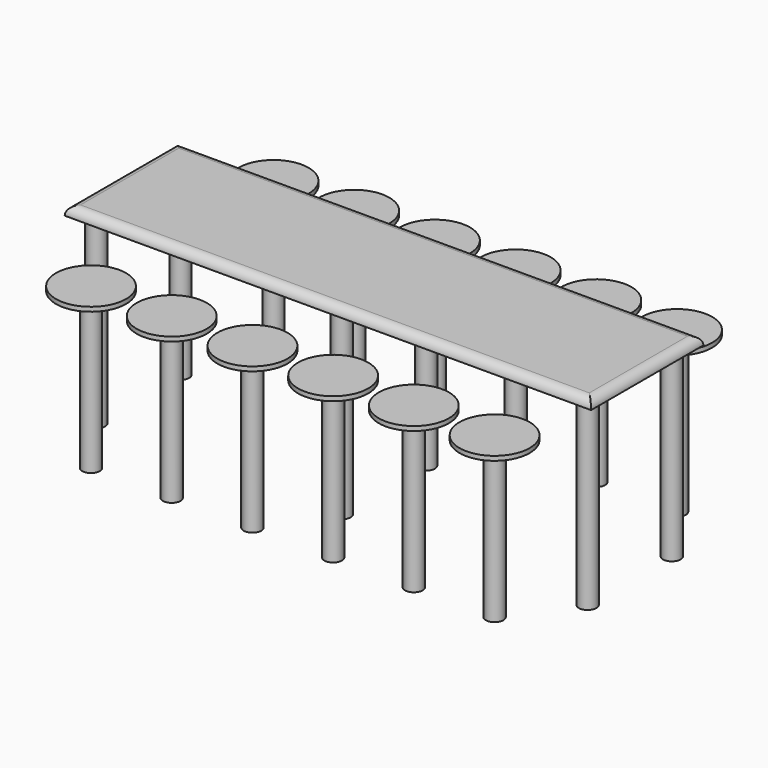
from build123d import *

# Parameters (mm, degrees)
F0_W      = 50
F0_H      = 1050
F1_DEPTH  = 800
F2_R      = 49.99999
F3_R      = 50
F4_DEPTH  = 900
F5_R      = 200
F6_DEPTH  = 12.5
F7_W      = 800
F7_H      = 1050
F8_DEPTH  = 3000.001
F9_R      = 50
F10_DEPTH = 1050


# Not quite as in the source:
# - a fillet or chamfer is up to 0.001 mm smaller than in the source, because OpenCascade refuses the exact size


with BuildPart() as f1:
    # F0 (on Front) → F1 (new body)
    with BuildSketch(Plane.XZ):
        Polygon((3000, 50), (0, 50), (0, 0), (50, 0), (1450, 0), (1500, 0), (2950, 0), (3000, 0), align=None)
        with Locations((25, -525)):
            Rectangle(F0_W, F0_H)
        with Locations((2975, -525)):
            Rectangle(F0_W, F0_H)
        with Locations((1475, -525)):
            Rectangle(F0_W, F0_H)
    extrude(amount=F1_DEPTH)

    # F2 (radius 50 in the source; OpenCascade refuses exactly that, so slightly less here)
    f2_edges = [f1.edges().sort_by_distance(p)[0] for p in [
        (0, -400, 50),
        (1500, -800, 50),
        (1500, 0, 50),
        (3000, -400, 50),
    ]]
    fillet(f2_edges, radius=F2_R)

    # F7 (on face) → F8 (cut, through all)
    with BuildSketch(Plane(origin=(0, 0, 0), x_dir=(0, -1, 0), z_dir=(-1, 0, 0))):
        with Locations((400, -525)):
            Rectangle(F7_W, F7_H)
    extrude(amount=-F8_DEPTH, mode=Mode.SUBTRACT)

    # F9 (on face) → F10 (join, through all)
    with BuildSketch(Plane(origin=(0, 0, 0), x_dir=(1, 0, 0), z_dir=(0, 0, -1))):
        with Locations((100, 700)):
            Circle(F9_R)
        with Locations((100, 100)):
            Circle(F9_R)
        with Locations((1500, 700)):
            Circle(F9_R)
        with Locations((1500, 100)):
            Circle(F9_R)
        with Locations((2900, 700)):
            Circle(F9_R)
        with Locations((2900, 100)):
            Circle(F9_R)
    extrude(amount=F10_DEPTH)


with BuildPart() as f4:
    # F3 (on face) → F4 (new body)
    with BuildSketch(Plane(origin=(0, 0, -1050), x_dir=(1, 0, 0), z_dir=(0, 0, -1))):
        with Locations((350, -250)):
            Circle(F3_R)
    extrude(amount=-F4_DEPTH)


with BuildPart() as f4b:
    # F3 (on face) → F4, piece 2 (new body)
    with BuildSketch(Plane(origin=(0, 0, -1050), x_dir=(1, 0, 0), z_dir=(0, 0, -1))):
        with Locations((350, 1050)):
            Circle(F3_R)
    extrude(amount=-F4_DEPTH)


with BuildPart() as f4c:
    # F3 (on face) → F4, piece 3 (new body)
    with BuildSketch(Plane(origin=(0, 0, -1050), x_dir=(1, 0, 0), z_dir=(0, 0, -1))):
        with Locations((810, -250)):
            Circle(F3_R)
    extrude(amount=-F4_DEPTH)


with BuildPart() as f4d:
    # F3 (on face) → F4, piece 4 (new body)
    with BuildSketch(Plane(origin=(0, 0, -1050), x_dir=(1, 0, 0), z_dir=(0, 0, -1))):
        with Locations((810, 1050)):
            Circle(F3_R)
    extrude(amount=-F4_DEPTH)


with BuildPart() as f4e:
    # F3 (on face) → F4, piece 5 (new body)
    with BuildSketch(Plane(origin=(0, 0, -1050), x_dir=(1, 0, 0), z_dir=(0, 0, -1))):
        with Locations((1270, -250)):
            Circle(F3_R)
    extrude(amount=-F4_DEPTH)


with BuildPart() as f4f:
    # F3 (on face) → F4, piece 6 (new body)
    with BuildSketch(Plane(origin=(0, 0, -1050), x_dir=(1, 0, 0), z_dir=(0, 0, -1))):
        with Locations((1270, 1050)):
            Circle(F3_R)
    extrude(amount=-F4_DEPTH)


with BuildPart() as f4g:
    # F3 (on face) → F4, piece 7 (new body)
    with BuildSketch(Plane(origin=(0, 0, -1050), x_dir=(1, 0, 0), z_dir=(0, 0, -1))):
        with Locations((1730, -250)):
            Circle(F3_R)
    extrude(amount=-F4_DEPTH)


with BuildPart() as f4h:
    # F3 (on face) → F4, piece 8 (new body)
    with BuildSketch(Plane(origin=(0, 0, -1050), x_dir=(1, 0, 0), z_dir=(0, 0, -1))):
        with Locations((1730, 1050)):
            Circle(F3_R)
    extrude(amount=-F4_DEPTH)


with BuildPart() as f4i:
    # F3 (on face) → F4, piece 9 (new body)
    with BuildSketch(Plane(origin=(0, 0, -1050), x_dir=(1, 0, 0), z_dir=(0, 0, -1))):
        with Locations((2190, -250)):
            Circle(F3_R)
    extrude(amount=-F4_DEPTH)


with BuildPart() as f4j:
    # F3 (on face) → F4, piece 10 (new body)
    with BuildSketch(Plane(origin=(0, 0, -1050), x_dir=(1, 0, 0), z_dir=(0, 0, -1))):
        with Locations((2190, 1050)):
            Circle(F3_R)
    extrude(amount=-F4_DEPTH)


with BuildPart() as f4k:
    # F3 (on face) → F4, piece 11 (new body)
    with BuildSketch(Plane(origin=(0, 0, -1050), x_dir=(1, 0, 0), z_dir=(0, 0, -1))):
        with Locations((2650, -250)):
            Circle(F3_R)
    extrude(amount=-F4_DEPTH)


with BuildPart() as f4l:
    # F3 (on face) → F4, piece 12 (new body)
    with BuildSketch(Plane(origin=(0, 0, -1050), x_dir=(1, 0, 0), z_dir=(0, 0, -1))):
        with Locations((2650, 1050)):
            Circle(F3_R)
    extrude(amount=-F4_DEPTH)


with BuildPart() as f6:
    # F5 (on face) → F6 (new body, symmetric)
    with BuildSketch(Plane.XY.offset(-150)):
        with Locations((350, 250)):
            Circle(F5_R)
    extrude(amount=F6_DEPTH, both=True)


with BuildPart() as f6b:
    # F5 (on face) → F6, piece 2 (new body, symmetric)
    with BuildSketch(Plane.XY.offset(-150)):
        with Locations((350, -1050)):
            Circle(F5_R)
    extrude(amount=F6_DEPTH, both=True)


with BuildPart() as f6c:
    # F5 (on face) → F6, piece 3 (new body, symmetric)
    with BuildSketch(Plane.XY.offset(-150)):
        with Locations((810, 250)):
            Circle(F5_R)
    extrude(amount=F6_DEPTH, both=True)


with BuildPart() as f6d:
    # F5 (on face) → F6, piece 4 (new body, symmetric)
    with BuildSketch(Plane.XY.offset(-150)):
        with Locations((810, -1050)):
            Circle(F5_R)
    extrude(amount=F6_DEPTH, both=True)


with BuildPart() as f6e:
    # F5 (on face) → F6, piece 5 (new body, symmetric)
    with BuildSketch(Plane.XY.offset(-150)):
        with Locations((1270, 250)):
            Circle(F5_R)
    extrude(amount=F6_DEPTH, both=True)


with BuildPart() as f6f:
    # F5 (on face) → F6, piece 6 (new body, symmetric)
    with BuildSketch(Plane.XY.offset(-150)):
        with Locations((1270, -1050)):
            Circle(F5_R)
    extrude(amount=F6_DEPTH, both=True)


with BuildPart() as f6g:
    # F5 (on face) → F6, piece 7 (new body, symmetric)
    with BuildSketch(Plane.XY.offset(-150)):
        with Locations((1730, 250)):
            Circle(F5_R)
    extrude(amount=F6_DEPTH, both=True)


with BuildPart() as f6h:
    # F5 (on face) → F6, piece 8 (new body, symmetric)
    with BuildSketch(Plane.XY.offset(-150)):
        with Locations((1730, -1050)):
            Circle(F5_R)
    extrude(amount=F6_DEPTH, both=True)


with BuildPart() as f6i:
    # F5 (on face) → F6, piece 9 (new body, symmetric)
    with BuildSketch(Plane.XY.offset(-150)):
        with Locations((2190, 250)):
            Circle(F5_R)
    extrude(amount=F6_DEPTH, both=True)


with BuildPart() as f6j:
    # F5 (on face) → F6, piece 10 (new body, symmetric)
    with BuildSketch(Plane.XY.offset(-150)):
        with Locations((2190, -1050)):
            Circle(F5_R)
    extrude(amount=F6_DEPTH, both=True)


with BuildPart() as f6k:
    # F5 (on face) → F6, piece 11 (new body, symmetric)
    with BuildSketch(Plane.XY.offset(-150)):
        with Locations((2650, 250)):
            Circle(F5_R)
    extrude(amount=F6_DEPTH, both=True)


with BuildPart() as f6l:
    # F5 (on face) → F6, piece 12 (new body, symmetric)
    with BuildSketch(Plane.XY.offset(-150)):
        with Locations((2650, -1050)):
            Circle(F5_R)
    extrude(amount=F6_DEPTH, both=True)


solid = Compound([f1.part, f4.part, f4b.part, f4c.part, f4d.part, f4e.part, f4f.part, f4g.part, f4h.part, f4i.part, f4j.part, f4k.part, f4l.part, f6.part, f6b.part, f6c.part, f6d.part, f6e.part, f6f.part, f6g.part, f6h.part, f6i.part, f6j.part, f6k.part, f6l.part])
